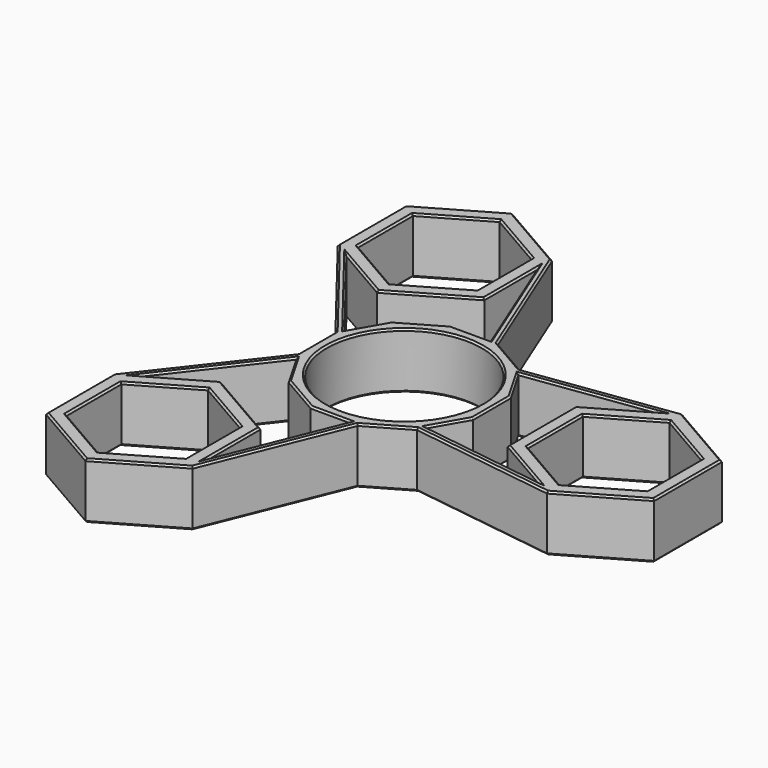
from build123d import *

# Parameters (mm, degrees)
F1_R     = 11.05
F2_DEPTH = 8
F3_SIZE  = 0.25


with BuildPart() as f2:
    # F1 (on Top) → F2 (new body)
    with BuildSketch(Plane.XY):
        Polygon((30, -12.0666206261), (40.45, -6.033310313), (40.45, 6.033310313), (30, 12.0666206261), (27.6919892048, 10.7340899722), (19.55, 6.033310313), (19.55, -6.033310313), (27.6919892048, -10.7340899722), align=None)
        Polygon((21.55, 4.8786097747), (30, 9.7572195493), (38.45, 4.8786097747), (38.45, -4.8786097747), (30, -9.7572195493), (21.55, -4.8786097747), align=None, mode=Mode.SUBTRACT)
        Polygon((9.1506350946, -9.1506350946), (30, -12.0666206261), (27.6919892048, -10.7340899722), (9.6900481732, -8.2163442363), align=None)
        Polygon((27.6919892048, 10.7340899722), (30, 12.0666206261), (9.1506350946, 9.1506350946), (9.6900481732, 8.2163442363), align=None)
        Polygon((3.3493649054, -12.5), (9.1506350946, -9.1506350946), (9.6900481732, -8.2163442363), (12.5, -3.3493649054), (12.5, 3.3493649054), (9.6900481732, 8.2163442363), (9.1506350946, 9.1506350946), (3.3493649054, 12.5), (2.2705387483, 12.5), (-3.3493649054, 12.5), (-9.1506350946, 9.1506350946), (-11.9605869214, 4.2836557637), (-12.5, 3.3493649054), (-12.5, -3.3493649054), (-11.9605869214, -4.2836557637), (-9.1506350946, -9.1506350946), (-3.3493649054, -12.5), (2.2705387483, -12.5), align=None)
        Circle(F1_R, mode=Mode.SUBTRACT)
        Polygon((-4.55, -32.0140724266), (3.3493649054, -12.5), (2.2705387483, -12.5), (-4.55, -29.3490111188), align=None)
        Polygon((2.2705387483, 12.5), (3.3493649054, 12.5), (-4.55, 32.0140724266), (-4.55, 29.3490111188), align=None)
        Polygon((-15, -38.0473827396), (-4.55, -32.0140724266), (-4.55, -29.3490111188), (-4.55, -19.9474518005), (-15, -13.9141414875), (-23.1419892048, -18.6149211466), (-25.45, -19.9474518005), (-25.45, -32.0140724266), align=None)
        Polygon((-23.45, -21.1021523389), (-15, -16.2235425642), (-6.55, -21.1021523389), (-6.55, -30.8593718882), (-15, -35.7379816628), (-23.45, -30.8593718882), align=None, mode=Mode.SUBTRACT)
        Polygon((-4.55, 29.3490111188), (-4.55, 32.0140724266), (-15, 38.0473827396), (-25.45, 32.0140724266), (-25.45, 19.9474518005), (-23.1419892048, 18.6149211466), (-15, 13.9141414875), (-4.55, 19.9474518005), align=None)
        Polygon((-6.55, 30.8593718882), (-6.55, 21.1021523389), (-15, 16.2235425642), (-23.45, 21.1021523389), (-23.45, 30.8593718882), (-15, 35.7379816628), align=None, mode=Mode.SUBTRACT)
        Polygon((-23.1419892048, -18.6149211466), (-11.9605869214, -4.2836557637), (-12.5, -3.3493649054), (-25.45, -19.9474518005), align=None)
        Polygon((-12.5, 3.3493649054), (-11.9605869214, 4.2836557637), (-23.1419892048, 18.6149211466), (-25.45, 19.9474518005), align=None)
    extrude(amount=F2_DEPTH)

    # F3
    f3_edges = [f2.edges().sort_by_distance(p)[0] for p in [
        (35.225, -9.049965, 0),
        (40.45, 0, 0),
        (35.225, 9.049965, 0),
        (19.575318, 10.608628, 0),
        (6.25, 10.825318, 0),
        (-0.600318, 22.257036, 0),
        (-9.775, 35.030728, 0),
        (-20.225, 35.030728, 0),
        (-25.45, 25.980762, 0),
        (-18.975, 11.648408, 0),
        (-12.5, 0, 0),
        (-18.975, -11.648408, 0),
        (-25.45, -25.980762, 0),
        (-20.225, -35.030728, 0),
        (-9.775, -35.030728, 0),
        (-0.600318, -22.257036, 0),
        (6.25, -10.825318, 0),
        (19.575318, -10.608628, 0),
        (-19.070995, 16.264531, 0),
        (-9.775, 16.930797, 0),
        (-4.55, 24.648231, 0),
        (-1.139731, 20.924506, 0),
        (-0.539413, 12.5, 0),
        (-6.25, 10.825318, 0),
        (-10.555611, 6.717145, 0),
        (-17.551288, 11.449288, 0),
        (-10.555611, -6.717145, 0),
        (-6.25, -10.825318, 0),
        (-0.539413, -12.5, 0),
        (-1.139731, -20.924506, 0),
        (-4.55, -24.648231, 0),
        (-9.775, -16.930797, 0),
        (-19.070995, -16.264531, 0),
        (-17.551288, -11.449288, 0),
        (18.691019, 9.475217, 0),
        (23.620995, 8.3837, 0),
        (19.55, 0, 0),
        (23.620995, -8.3837, 0),
        (18.691019, -9.475217, 0),
        (11.095024, -5.782855, 0),
        (12.5, 0, 0),
        (11.095024, 5.782855, 0),
        (25.775, -7.317915, 0),
        (21.55, 0, 0),
        (25.775, 7.317915, 0),
        (34.225, 7.317915, 0),
        (38.45, 0, 0),
        (34.225, -7.317915, 0),
        (-11.05, 0, 0),
        (-23.45, -25.980762, 0),
        (-19.225, -18.662847, 0),
        (-10.775, -18.662847, 0),
        (-6.55, -25.980762, 0),
        (-10.775, -33.298677, 0),
        (-19.225, -33.298677, 0),
        (-19.225, 33.298677, 0),
        (-10.775, 33.298677, 0),
        (-6.55, 25.980762, 0),
        (-10.775, 18.662847, 0),
        (-19.225, 18.662847, 0),
        (-23.45, 25.980762, 0),
        (35.225, -9.049965, 8),
        (40.45, 0, 8),
        (35.225, 9.049965, 8),
        (19.575318, 10.608628, 8),
        (6.25, 10.825318, 8),
        (-0.600318, 22.257036, 8),
        (-9.775, 35.030728, 8),
        (-20.225, 35.030728, 8),
        (-25.45, 25.980762, 8),
        (-18.975, 11.648408, 8),
        (-12.5, 0, 8),
        (-18.975, -11.648408, 8),
        (-25.45, -25.980762, 8),
        (-20.225, -35.030728, 8),
        (-9.775, -35.030728, 8),
        (-0.600318, -22.257036, 8),
        (6.25, -10.825318, 8),
        (19.575318, -10.608628, 8),
        (-19.070995, 16.264531, 8),
        (-9.775, 16.930797, 8),
        (-4.55, 24.648231, 8),
        (-1.139731, 20.924506, 8),
        (-0.539413, 12.5, 8),
        (-6.25, 10.825318, 8),
        (-10.555611, 6.717145, 8),
        (-17.551288, 11.449288, 8),
        (-10.555611, -6.717145, 8),
        (-6.25, -10.825318, 8),
        (-0.539413, -12.5, 8),
        (-1.139731, -20.924506, 8),
        (-4.55, -24.648231, 8),
        (-9.775, -16.930797, 8),
        (-19.070995, -16.264531, 8),
        (-17.551288, -11.449288, 8),
        (18.691019, 9.475217, 8),
        (23.620995, 8.3837, 8),
        (19.55, 0, 8),
        (23.620995, -8.3837, 8),
        (18.691019, -9.475217, 8),
        (11.095024, -5.782855, 8),
        (12.5, 0, 8),
        (11.095024, 5.782855, 8),
        (25.775, -7.317915, 8),
        (21.55, 0, 8),
        (25.775, 7.317915, 8),
        (34.225, 7.317915, 8),
        (38.45, 0, 8),
        (34.225, -7.317915, 8),
        (-11.05, 0, 8),
        (-23.45, -25.980762, 8),
        (-19.225, -18.662847, 8),
        (-10.775, -18.662847, 8),
        (-6.55, -25.980762, 8),
        (-10.775, -33.298677, 8),
        (-19.225, -33.298677, 8),
        (-19.225, 33.298677, 8),
        (-10.775, 33.298677, 8),
        (-6.55, 25.980762, 8),
        (-10.775, 18.662847, 8),
        (-19.225, 18.662847, 8),
        (-23.45, 25.980762, 8),
    ]]
    chamfer(f3_edges, length=F3_SIZE)


solid = f2.part
